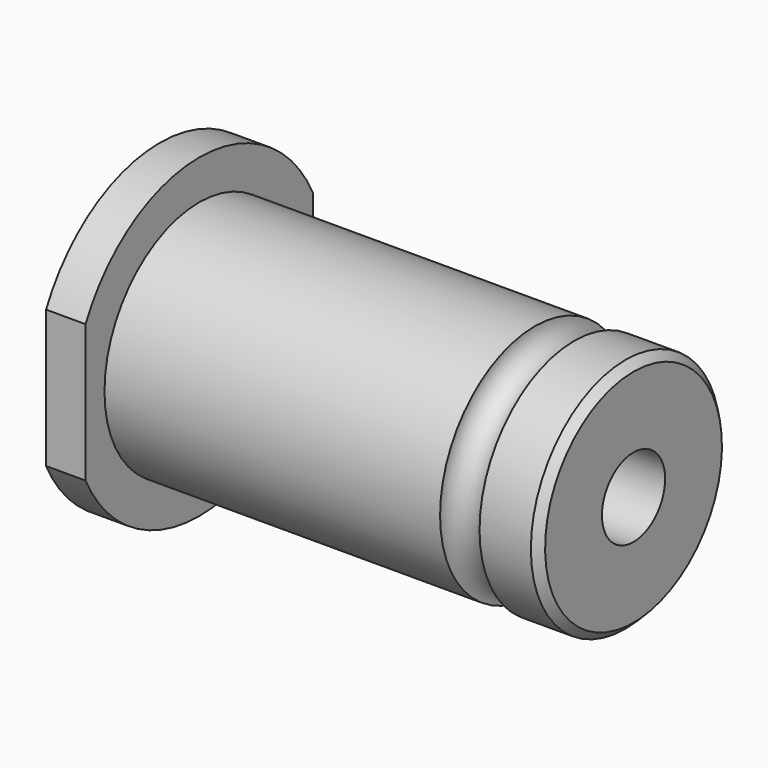
from build123d import *

# Parameters (mm, degrees)
F2_R     = 5
F3_DEPTH = 60.001
F4_SIZE  = 1
F5_R     = 2.5
F8_DEPTH = 5


# Not quite as in the source:
# - a pattern or mirror of a feature is missing from the dataset's text; its kind, count and spacing are read off the source's solid


with BuildPart() as f1:
    # F0 (on Front) → F1 (revolve)
    with BuildSketch(Plane.XZ):
        Polygon((0, 20), (0, 0), (60, 0), (60, 15), (5, 15), (5, 20), align=None)
    revolve(axis=Axis((31.1737104983, 0, 0), (-1, 0, 0)))

    # F2 (on face) → F3 (cut, through all)
    with BuildSketch(Plane.YZ.offset(60)):
        Circle(F2_R)
    extrude(amount=-F3_DEPTH, mode=Mode.SUBTRACT)

    # F4
    f4_edges = [f1.edges().sort_by_distance(p)[0] for p in [
        (60, 0, -15),
    ]]
    chamfer(f4_edges, length=F4_SIZE)

    # F5 (on Front) → F6 (revolve, cut)
    with BuildSketch(Plane.XZ):
        with Locations((50, 15)):
            Circle(F5_R)
    revolve(axis=Axis((31.1737104983, 0, 0), (-1, 0, 0)), mode=Mode.SUBTRACT)

    # F7 (on face) → F8 (cut, through all)
    with BuildSketch(Plane(origin=(0, 0, 0), x_dir=(0, -1, 0), z_dir=(-1, 0, 0))):
        with BuildLine():
            ThreePointArc((18, -8.7177978871), (19.4935886896, -4.472135955), (20, 0))
            ThreePointArc((20, 0), (19.4935886896, 4.472135955), (18, 8.7177978871))
            Line((18, 8.7177978871), (18, -8.7177978871))
        make_face()
    f8 = extrude(amount=-F8_DEPTH, mode=Mode.SUBTRACT)

    # F8_copies: F8 across plane
    add(f8.mirror(Plane.ZX), mode=Mode.SUBTRACT)


solid = f1.part
